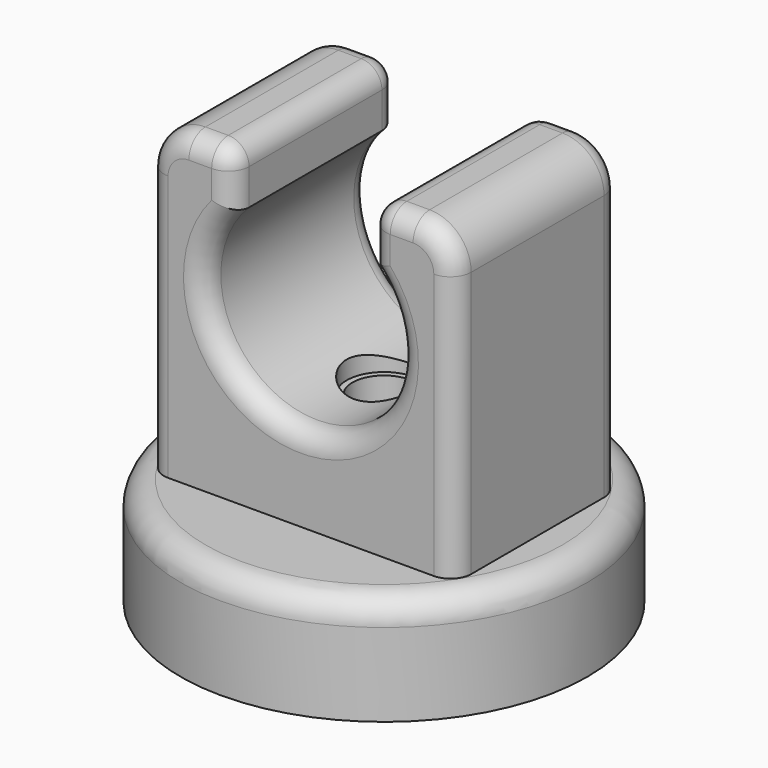
from build123d import *

# Parameters (mm, degrees)
F0_R          = 24.5
F1_DEPTH      = 13
F2_W          = 37
F2_H          = 25
F3_DEPTH      = 37
F5_R          = 3.8
F6_DEPTH      = 60
F7_R          = 11.65
F8_DEPTH      = 40
F9_W          = 16.5
F9_H          = 25
F10_DEPTH     = 10
F11_R         = 4.5
F12_DEPTH     = 28
F13_T1_DEPTH  = 14
F13_T3_DEPTH  = 14
F13_T5_DEPTH  = 10.5744301109
F13_T7_DEPTH  = 20
F13_S11_W     = 2.5
F13_S11_H     = 2.5
F13_T12_DEPTH = 2.5
F13_S17_W     = 2.5
F13_S17_H     = 2.5
F13_T18_DEPTH = 2.5
F13_S23_W     = 2.5
F13_S23_H     = 2.5
F13_T24_DEPTH = 2.5
F13_S29_W     = 2.5
F13_S29_H     = 2.5
F13_T30_DEPTH = 2.5
F13_T36_DEPTH = 49.44
F13_T41_DEPTH = 49.44
F13_T46_DEPTH = 49.44
F13_T51_DEPTH = 49.44
F13_T54_ANGLE = 331.528720339
F13_T56_ANGLE = 331.528720339
F14_T1_DEPTH  = 24.9999999998
F14_T4_ANGLE  = 90
F14_T6_ANGLE  = 90
F14_T8_ANGLE  = 90
F14_T10_ANGLE = 90


# Not quite as in the source:
# - a fillet or chamfer that OpenCascade refuses, or shapes differently, is made with other operations: its cross-section is extruded or revolved along the edge and cut away or added


with BuildPart() as f1:
    # F0 (on Top) → F1 (new body)
    with BuildSketch(Plane.XY):
        Circle(F0_R)
    extrude(amount=F1_DEPTH)

    # F2 (on face) → F3 (join)
    with BuildSketch(Plane.XY.offset(13)):
        Rectangle(F2_W, F2_H)
    extrude(amount=F3_DEPTH)

    # F4: fillet of radius 3 on 1 edges, made by hand

    # F4_s1 → F4_t2 (revolve, cut)
    with BuildSketch(Plane.XZ):
        with BuildLine():
            ThreePointArc((24.5, 10), (23.6213203436, 12.1213203436), (21.5, 13))
            Line((21.5, 13), (21.5, 13.06))
            Line((21.5, 13.06), (24.56, 13.06))
            Line((24.56, 13.06), (24.56, 10))
            Line((24.56, 10), (24.5, 10))
        make_face()
    revolve(axis=Axis((0, 0, 13), (0, 0, 1)), mode=Mode.SUBTRACT)

    # F5 (on face) → F6 (cut)
    with BuildSketch(Plane.XY.offset(50)):
        Circle(F5_R)
    extrude(amount=-F6_DEPTH, mode=Mode.SUBTRACT)

    # F7 (on face) → F8 (cut)
    with BuildSketch(Plane.XZ.offset(12.5)):
        with Locations((0, 34.95)):
            Circle(F7_R)
    extrude(amount=-F8_DEPTH, mode=Mode.SUBTRACT)

    # F9 (on face) → F10 (cut)
    with BuildSketch(Plane.XY.offset(50)):
        Rectangle(F9_W, F9_H)
    extrude(amount=-F10_DEPTH, mode=Mode.SUBTRACT)

    # F11 (on face) → F12 (cut)
    with BuildSketch(Plane.XY.offset(50)):
        Circle(F11_R)
    extrude(amount=-F12_DEPTH, mode=Mode.SUBTRACT)

    # F13: fillet of radius 2.5 on 16 edges, made by hand

    # F13_s2 → F13_t1 (cut)
    with BuildSketch(Plane.YZ.offset(-24.75)):
        with BuildLine():
            ThreePointArc((-12.5, 47.5), (-11.767766953, 49.267766953), (-10, 50))
            Line((-10, 50), (-12.5, 50))
            Line((-12.5, 50), (-12.5, 47.5))
        make_face()
        with BuildLine():
            ThreePointArc((12.5, 47.5), (11.767766953, 49.267766953), (10, 50))
            Line((10, 50), (12.5, 50))
            Line((12.5, 50), (12.5, 47.5))
        make_face()
    extrude(amount=F13_T1_DEPTH, mode=Mode.SUBTRACT)

    # F13_s4 → F13_t3 (cut)
    with BuildSketch(Plane.YZ.offset(10.75)):
        with BuildLine():
            ThreePointArc((-12.5, 47.5), (-11.767766953, 49.267766953), (-10, 50))
            Line((-10, 50), (-12.5, 50))
            Line((-12.5, 50), (-12.5, 47.5))
        make_face()
        with BuildLine():
            ThreePointArc((12.5, 47.5), (11.767766953, 49.267766953), (10, 50))
            Line((10, 50), (12.5, 50))
            Line((12.5, 50), (12.5, 47.5))
        make_face()
    extrude(amount=F13_T3_DEPTH, mode=Mode.SUBTRACT)

    # F13_s6 → F13_t5 (cut)
    with BuildSketch(Plane.XY.offset(36.9255698891)):
        with BuildLine():
            ThreePointArc((-10.75, -12.5), (-8.982233047, -11.767766953), (-8.25, -10))
            Line((-8.25, -10), (-8.25, -12.5))
            Line((-8.25, -12.5), (-10.75, -12.5))
        make_face()
        with BuildLine():
            ThreePointArc((10.75, -12.5), (8.982233047, -11.767766953), (8.25, -10))
            Line((8.25, -10), (8.25, -12.5))
            Line((8.25, -12.5), (10.75, -12.5))
        make_face()
        with BuildLine():
            ThreePointArc((10.75, 12.5), (8.982233047, 11.767766953), (8.25, 10))
            Line((8.25, 10), (8.25, 12.5))
            Line((8.25, 12.5), (10.75, 12.5))
        make_face()
        with BuildLine():
            ThreePointArc((-10.75, 12.5), (-8.982233047, 11.767766953), (-8.25, 10))
            Line((-8.25, 10), (-8.25, 12.5))
            Line((-8.25, 12.5), (-10.75, 12.5))
        make_face()
    extrude(amount=F13_T5_DEPTH, mode=Mode.SUBTRACT)

    # F13_s8 → F13_t7 (cut)
    with BuildSketch(Plane.XZ.offset(-10)):
        with BuildLine():
            ThreePointArc((10.75, 50), (8.982233047, 49.267766953), (8.25, 47.5))
            Line((8.25, 47.5), (8.25, 50))
            Line((8.25, 50), (10.75, 50))
        make_face()
        with BuildLine():
            ThreePointArc((-8.25, 47.5), (-8.982233047, 49.267766953), (-10.75, 50))
            Line((-10.75, 50), (-8.25, 50))
            Line((-8.25, 50), (-8.25, 47.5))
        make_face()
    extrude(amount=F13_T7_DEPTH, mode=Mode.SUBTRACT)


with BuildPart() as f13_tool10:
    # F13_s11 → F13_t12 (new body)
    with BuildSketch(Plane.YZ.offset(-10.75)):
        with Locations((-11.25, 48.75)):
            Rectangle(F13_S11_W, F13_S11_H)
    extrude(amount=F13_T12_DEPTH)

    # F13_s13 → F13_t14 (revolve, cut)
    with BuildSketch(Plane(origin=(-10.75, -10, 47.5), x_dir=(0, 0.7071067812, -0.7071067812), z_dir=(0, -0.7071067812, -0.7071067812))):
        with BuildLine():
            ThreePointArc((0, -2.5), (2.5, 0), (0, 2.5))
            Line((0, 2.5), (0, -2.5))
        make_face()
    revolve(axis=Axis((-10.75, -10, 47.5), (1, 0, 0)), mode=Mode.SUBTRACT)


with BuildPart() as f1_1:
    add(f1.part)

    # F13_t9: cut F13_tool10
    add(f13_tool10.part, mode=Mode.SUBTRACT)


with BuildPart() as f13_tool16:
    # F13_s17 → F13_t18 (new body)
    with BuildSketch(Plane.XZ.offset(10)):
        with Locations((9.5, 48.75)):
            Rectangle(F13_S17_W, F13_S17_H)
    extrude(amount=F13_T18_DEPTH)

    # F13_s19 → F13_t20 (revolve, cut)
    with BuildSketch(Plane(origin=(10.75, -10, 47.5), x_dir=(0.7071067812, 0, -0.7071067812), z_dir=(-0.7071067812, 0, -0.7071067812))):
        with BuildLine():
            ThreePointArc((0, -2.5), (2.5, 0), (0, 2.5))
            Line((0, 2.5), (0, -2.5))
        make_face()
    revolve(axis=Axis((10.75, -10, 47.5), (0, -1, 0)), mode=Mode.SUBTRACT)


with BuildPart() as f1_2:
    add(f1_1.part)

    # F13_t15: cut F13_tool16
    add(f13_tool16.part, mode=Mode.SUBTRACT)


with BuildPart() as f13_tool22:
    # F13_s23 → F13_t24 (new body)
    with BuildSketch(Plane.YZ.offset(-10.75)):
        with Locations((11.25, 48.75)):
            Rectangle(F13_S23_W, F13_S23_H)
    extrude(amount=F13_T24_DEPTH)

    # F13_s25 → F13_t26 (revolve, cut)
    with BuildSketch(Plane(origin=(-10.75, 10, 47.5), x_dir=(0, -0.7071067812, -0.7071067812), z_dir=(0, -0.7071067812, 0.7071067812))):
        with BuildLine():
            ThreePointArc((0, -2.5), (2.5, 0), (0, 2.5))
            Line((0, 2.5), (0, -2.5))
        make_face()
    revolve(axis=Axis((-10.75, 10, 47.5), (1, 0, 0)), mode=Mode.SUBTRACT)


with BuildPart() as f1_3:
    add(f1_2.part)

    # F13_t21: cut F13_tool22
    add(f13_tool22.part, mode=Mode.SUBTRACT)


with BuildPart() as f13_tool28:
    # F13_s29 → F13_t30 (new body)
    with BuildSketch(Plane.YZ.offset(10.75)):
        with Locations((11.25, 48.75)):
            Rectangle(F13_S29_W, F13_S29_H)
    extrude(amount=-F13_T30_DEPTH)

    # F13_s31 → F13_t32 (revolve, cut)
    with BuildSketch(Plane(origin=(10.75, 10, 47.5), x_dir=(0, -0.7071067812, -0.7071067812), z_dir=(0, 0.7071067812, -0.7071067812))):
        with BuildLine():
            ThreePointArc((0, -2.5), (2.5, 0), (0, 2.5))
            Line((0, 2.5), (0, -2.5))
        make_face()
    revolve(axis=Axis((10.75, 10, 47.5), (-1, 0, 0)), mode=Mode.SUBTRACT)


with BuildPart() as f1_4:
    add(f1_3.part)

    # F13_t27: cut F13_tool28
    add(f13_tool28.part, mode=Mode.SUBTRACT)


with BuildPart() as f13_tool34:
    # F13_s35 → F13_t36 (new body)
    with BuildSketch(Plane.XY.offset(6.81)):
        with BuildLine():
            ThreePointArc((18.5, 10), (17.767766953, 11.767766953), (16, 12.5))
            Line((16, 12.5), (18.5, 12.5))
            Line((18.5, 12.5), (18.5, 10))
        make_face()
    extrude(amount=F13_T36_DEPTH)

    split(bisect_by=Plane.XY.offset(13), keep=Keep.TOP)


with BuildPart() as f1_5:
    add(f1_4.part)

    # F13_t33: cut F13_tool34
    add(f13_tool34.part, mode=Mode.SUBTRACT)


with BuildPart() as f13_tool39:
    # F13_s40 → F13_t41 (new body)
    with BuildSketch(Plane.XY.offset(6.81)):
        with BuildLine():
            ThreePointArc((-16, 12.5), (-17.767766953, 11.767766953), (-18.5, 10))
            Line((-18.5, 10), (-18.5, 12.5))
            Line((-18.5, 12.5), (-16, 12.5))
        make_face()
    extrude(amount=F13_T41_DEPTH)

    split(bisect_by=Plane.XY.offset(13), keep=Keep.TOP)


with BuildPart() as f1_6:
    add(f1_5.part)

    # F13_t38: cut F13_tool39
    add(f13_tool39.part, mode=Mode.SUBTRACT)


with BuildPart() as f13_tool44:
    # F13_s45 → F13_t46 (new body)
    with BuildSketch(Plane.XY.offset(6.81)):
        with BuildLine():
            ThreePointArc((18.5, -10), (17.767766953, -11.767766953), (16, -12.5))
            Line((16, -12.5), (18.5, -12.5))
            Line((18.5, -12.5), (18.5, -10))
        make_face()
    extrude(amount=F13_T46_DEPTH)

    split(bisect_by=Plane.XY.offset(13), keep=Keep.TOP)


with BuildPart() as f1_7:
    add(f1_6.part)

    # F13_t43: cut F13_tool44
    add(f13_tool44.part, mode=Mode.SUBTRACT)


with BuildPart() as f13_tool49:
    # F13_s50 → F13_t51 (new body)
    with BuildSketch(Plane.XY.offset(6.81)):
        with BuildLine():
            ThreePointArc((-18.5, -10), (-17.767766953, -11.767766953), (-16, -12.5))
            Line((-16, -12.5), (-18.5, -12.5))
            Line((-18.5, -12.5), (-18.5, -10))
        make_face()
    extrude(amount=F13_T51_DEPTH)

    split(bisect_by=Plane.XY.offset(13), keep=Keep.TOP)


with BuildPart() as f1_8:
    add(f1_7.part)

    # F13_t48: cut F13_tool49
    add(f13_tool49.part, mode=Mode.SUBTRACT)

    # F13_s53 → F13_t54 (revolve, cut)
    with BuildSketch(Plane(origin=(-8.3306502048, 0, 2.1134931675), x_dir=(0, 1, 0), z_dir=(-0.9692925732, 0, 0.2459103648))):
        with BuildLine():
            ThreePointArc((12.5, -48.0267754339), (11.767766953, -46.2590084809), (10, -45.5267754339))
            Line((10, -45.5267754339), (12.5, -45.5267754339))
            Line((12.5, -45.5267754339), (12.5, -48.0267754339))
        make_face()
    revolve(axis=Axis((0, 12.5, 34.95), (0, 1, 0)), revolution_arc=F13_T54_ANGLE, mode=Mode.SUBTRACT)

    # F13_s55 → F13_t56 (revolve, cut)
    with BuildSketch(Plane(origin=(8.3306502048, 0, 2.1134931675), x_dir=(0, 1, 0), z_dir=(0.9692925732, 0, 0.2459103648))):
        with BuildLine():
            ThreePointArc((-12.5, 48.0267754339), (-11.767766953, 46.2590084809), (-10, 45.5267754339))
            Line((-10, 45.5267754339), (-12.5, 45.5267754339))
            Line((-12.5, 45.5267754339), (-12.5, 48.0267754339))
        make_face()
    revolve(axis=Axis((0, -12.5, 34.95), (0, -1, 0)), revolution_arc=F13_T56_ANGLE, mode=Mode.SUBTRACT)

    # F14: fillet of radius 5 on 2 edges, made by hand

    # F14_s2 → F14_t1 (cut)
    with BuildSketch(Plane.XZ.offset(-12.4999999999)):
        with BuildLine():
            ThreePointArc((18.5, 45), (17.0355339059, 48.5355339059), (13.5, 50))
            Line((13.5, 50), (18.5, 50))
            Line((18.5, 50), (18.5, 45))
        make_face()
        with BuildLine():
            ThreePointArc((-18.5, 45), (-17.0355339059, 48.5355339059), (-13.5, 50))
            Line((-13.5, 50), (-18.5, 50))
            Line((-18.5, 50), (-18.5, 45))
        make_face()
    extrude(amount=F14_T1_DEPTH, mode=Mode.SUBTRACT)

    # F14_s3 → F14_t4 (revolve, cut)
    with BuildSketch(Plane.XY.offset(45)):
        with BuildLine():
            ThreePointArc((-16.0000000001, 12.5), (-17.767766953, 11.767766953), (-18.5, 10.0000000001))
            Line((-18.5, 10.0000000001), (-18.5, 12.5))
            Line((-18.5, 12.5), (-16.0000000001, 12.5))
        make_face()
    revolve(axis=Axis((-13.5, 12.5, 45), (0, 1, 0)), revolution_arc=F14_T4_ANGLE, mode=Mode.SUBTRACT)

    # F14_s5 → F14_t6 (revolve, cut)
    with BuildSketch(Plane.YZ.offset(-13.5)):
        with BuildLine():
            ThreePointArc((-12.5, 47.5000000001), (-11.767766953, 49.267766953), (-10.0000000001, 50))
            Line((-10.0000000001, 50), (-12.5, 50))
            Line((-12.5, 50), (-12.5, 47.5000000001))
        make_face()
    revolve(axis=Axis((-13.5, -12.5, 45), (0, -1, 0)), revolution_arc=F14_T6_ANGLE, mode=Mode.SUBTRACT)

    # F14_s7 → F14_t8 (revolve, cut)
    with BuildSketch(Plane.XY.offset(45)):
        with BuildLine():
            ThreePointArc((16.0000000001, -12.5), (17.767766953, -11.767766953), (18.5, -10.0000000001))
            Line((18.5, -10.0000000001), (18.5, -12.5))
            Line((18.5, -12.5), (16.0000000001, -12.5))
        make_face()
    revolve(axis=Axis((13.5, -12.5, 45), (0, -1, 0)), revolution_arc=F14_T8_ANGLE, mode=Mode.SUBTRACT)

    # F14_s9 → F14_t10 (revolve, cut)
    with BuildSketch(Plane.YZ.offset(13.5)):
        with BuildLine():
            ThreePointArc((12.5, 47.5000000001), (11.767766953, 49.267766953), (10.0000000001, 50))
            Line((10.0000000001, 50), (12.5, 50))
            Line((12.5, 50), (12.5, 47.5000000001))
        make_face()
    revolve(axis=Axis((13.5, 12.5, 45), (0, 1, 0)), revolution_arc=F14_T10_ANGLE, mode=Mode.SUBTRACT)


solid = f1_8.part
